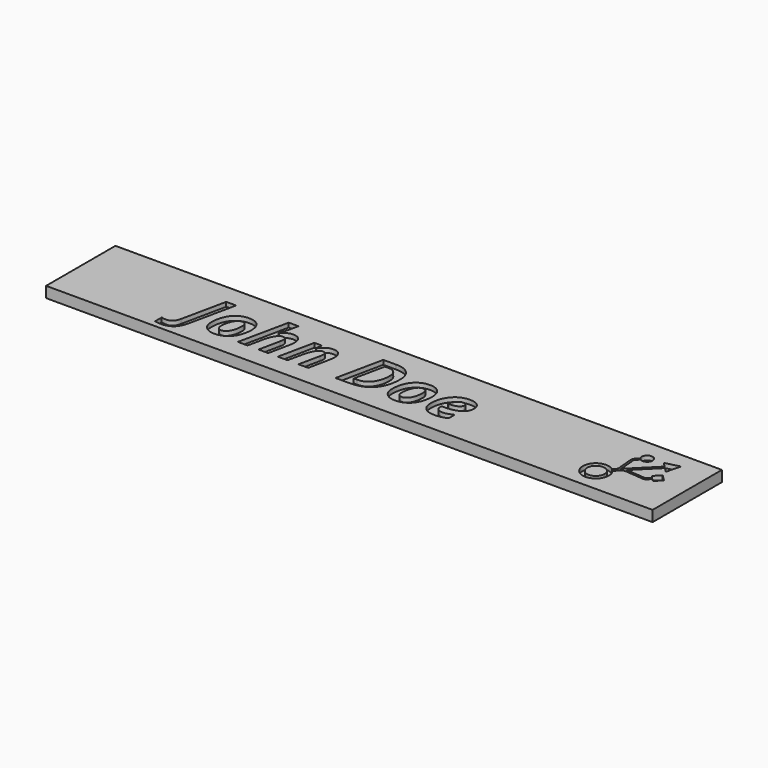
from build123d import *

# Parameters (mm, degrees)
F0_W         = 355.6
F0_H         = 50.8
F1_DEPTH     = 6.35
F2_TEXT_SIZE = 38.8055555556
F3_DEPTH     = 2.54
F5_DEPTH     = 2.54


# Not quite as in the source:
# - Text() gives the source's letters only with a copy of the font that has no kerning and outlines rounded to 1/6400 em; it was checked with that copy


with BuildPart() as f1:
    # F0 (on Top) → F1 (new body)
    with BuildSketch(Plane.XY):
        with Locations((177.8, 25.4)):
            Rectangle(F0_W, F0_H)
    extrude(amount=F1_DEPTH)

    # F2 (on face) → F3 (cut)
    with BuildSketch(Plane.XY.offset(6.35)):
        with Locations((67.0277777778, 11.43)):
            Text('John Doe', F2_TEXT_SIZE, font='Open Sans', font_style=FontStyle.BOLDITALIC, text_align=(TextAlign.LEFT, TextAlign.BOTTOM))
    extrude(amount=-F3_DEPTH, mode=Mode.SUBTRACT)

    # F4 (on face) → F5 (cut)
    with BuildSketch(Plane.XY.offset(6.35)):
        with BuildLine():
            ThreePointArc((315.3152886086, 16.8780527517), (315.9959295358, 15.4942594707), (316.23, 13.97))
            ThreePointArc((316.23, 13.97), (306.6455961561, 11.6212245721), (314.0580527517, 18.1352886086))
            Line((314.0580527517, 18.1352886086), (315.8727407308, 19.9499765877))
            ThreePointArc((315.8727407308, 19.9499765877), (304.2924609236, 10.6475674852), (318.77, 13.97))
            ThreePointArc((318.77, 13.97), (318.3483269445, 16.4696978219), (317.1299765877, 18.6927407308))
            Line((317.1299765877, 18.6927407308), (315.3152886086, 16.8780527517))
        make_face()
        with BuildLine():
            ThreePointArc((314.7421024484, 17.5621024484), (315.0437462681, 17.232689075), (315.3152886086, 16.8780527517))
            Line((315.3152886086, 16.8780527517), (317.1299765877, 18.6927407308))
            ThreePointArc((317.1299765877, 18.6927407308), (316.84379399, 19.0341001175), (316.5381536726, 19.3581536726))
            Line((316.5381536726, 19.3581536726), (314.7421024484, 17.5621024484))
        make_face()
        with BuildLine():
            Line((315.8727407308, 19.9499765877), (314.0580527517, 18.1352886086))
            ThreePointArc((314.0580527517, 18.1352886086), (314.412689075, 17.8637462681), (314.7421024484, 17.5621024484))
            Line((314.7421024484, 17.5621024484), (316.5381536726, 19.3581536726))
            ThreePointArc((316.5381536726, 19.3581536726), (316.2141001175, 19.66379399), (315.8727407308, 19.9499765877))
        make_face()
        with BuildLine():
            ThreePointArc((316.5381536726, 19.3581536726), (316.84379399, 19.0341001175), (317.1299765877, 18.6927407308))
            Line((317.1299765877, 18.6927407308), (319.9213616093, 21.4841257523))
            ThreePointArc((319.9213616093, 21.4841257523), (320.8486816694, 22.0748937849), (321.93878842, 22.2184090612))
            Line((321.93878842, 22.2184090612), (332.6786730213, 21.2787909111))
            ThreePointArc((332.6786730213, 21.2787909111), (333.7687797719, 21.4223061874), (334.6960998321, 22.01307422))
            Line((334.6960998321, 22.01307422), (336.4729615818, 23.7899359697))
            Line((336.4729615818, 23.7899359697), (335.5749359697, 24.6879615818))
            Line((335.5749359697, 24.6879615818), (333.79807422, 22.9110998321))
            ThreePointArc((333.79807422, 22.9110998321), (333.3344141899, 22.6157158158), (332.7893608146, 22.5439581776))
            Line((332.7893608146, 22.5439581776), (321.7660073724, 23.5083766379))
            Line((321.7660073724, 23.5083766379), (334.1394556699, 35.8818249354))
            Line((334.1394556699, 35.8818249354), (333.6006403027, 36.4206403027))
            Line((333.6006403027, 36.4206403027), (316.5381536726, 19.3581536726))
        make_face()
        with BuildLine():
            Line((316.8680745281, 20.945310385), (315.8727407308, 19.9499765877))
            ThreePointArc((315.8727407308, 19.9499765877), (316.2141001175, 19.66379399), (316.5381536726, 19.3581536726))
            Line((316.5381536726, 19.3581536726), (333.6006403027, 36.4206403027))
            Line((333.6006403027, 36.4206403027), (333.0618249354, 36.9594556699))
            Line((333.0618249354, 36.9594556699), (318.8923254137, 22.7899561482))
            Line((318.8923254137, 22.7899561482), (318.0300786876, 32.6454813246))
            ThreePointArc((318.0300786876, 32.6454813246), (318.1018363258, 33.1905346999), (318.3972203421, 33.65419473))
            Line((318.3972203421, 33.65419473), (320.1943082804, 35.4512826683))
            ThreePointArc((320.1943082804, 35.4512826683), (319.6999359697, 35.8549359697), (319.2962826683, 36.3493082804))
            Line((319.2962826683, 36.3493082804), (317.49919473, 34.5522203421))
            ThreePointArc((317.49919473, 34.5522203421), (316.9084266974, 33.6249002819), (316.764911421, 32.5347935313))
            Line((316.764911421, 32.5347935313), (317.602357837, 22.9627371958))
            ThreePointArc((317.602357837, 22.9627371958), (317.4588425607, 21.8726304452), (316.8680745281, 20.945310385))
        make_face()
        Polygon((333.0618249354, 36.9594556699), (333.6006403027, 36.4206403027), (334.1394556699, 35.8818249354), (336.711492276, 33.3097883293), (338.9887939753, 41.8087939753), (330.4897883293, 39.531492276), align=None)
        Polygon((338.2690128061, 25.5859871939), (336.4729615818, 23.7899359697), (337.82, 22.4428975516), (341.4121024484, 26.035), (337.82, 29.6271024484), (334.2278975516, 26.035), (335.5749359697, 24.6879615818), (337.3709871939, 26.4840128061), (337.82, 26.035), align=None)
        Polygon((335.5749359697, 24.6879615818), (336.4729615818, 23.7899359697), (338.2690128061, 25.5859871939), (337.82, 26.035), (337.3709871939, 26.4840128061), align=None)
        with BuildLine():
            Line((321.4959871939, 38.5490128061), (319.2962826683, 36.3493082804))
            ThreePointArc((319.2962826683, 36.3493082804), (319.6999359697, 35.8549359697), (320.1943082804, 35.4512826683))
            Line((320.1943082804, 35.4512826683), (322.3940128061, 37.6509871939))
            Line((322.3940128061, 37.6509871939), (321.945, 38.1))
            Line((321.945, 38.1), (321.4959871939, 38.5490128061))
        make_face()
        with BuildLine():
            ThreePointArc((325.12, 38.1), (321.0309574758, 41.1405840334), (319.2962826683, 36.3493082804))
            Line((319.2962826683, 36.3493082804), (321.4959871939, 38.5490128061))
            Line((321.4959871939, 38.5490128061), (321.945, 38.1))
            Line((321.945, 38.1), (322.3940128061, 37.6509871939))
            Line((322.3940128061, 37.6509871939), (320.1943082804, 35.4512826683))
            ThreePointArc((320.1943082804, 35.4512826683), (323.4486919216, 35.3036567441), (325.12, 38.1))
        make_face()
    extrude(amount=-F5_DEPTH, mode=Mode.SUBTRACT)


solid = f1.part
